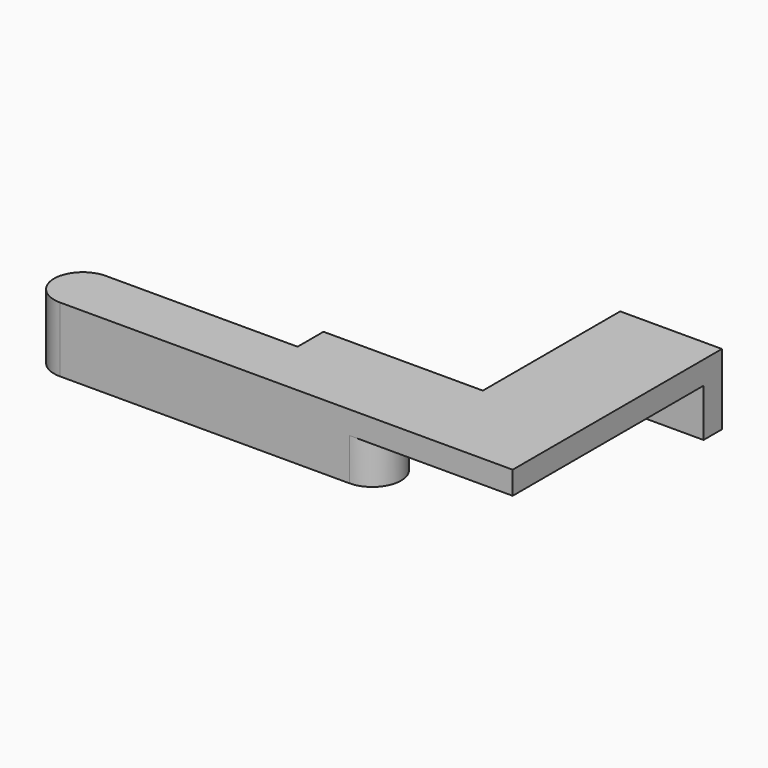
from build123d import *

# Parameters (mm, degrees)
F1_DEPTH = 4.6482
F2_W     = 11.2398419182
F2_H     = 2.54
F3_DEPTH = 2.54
F4_DEPTH = 5.2832


with BuildPart() as f1:
    # F0 (on Top) → F1 (new body)
    with BuildSketch(Plane.XY):
        with BuildLine():
            ThreePointArc((0, 6.35), (-3.175, 3.175), (0, 0))
            Line((0, 0), (31.9786, 0))
            ThreePointArc((31.9786, 0), (35.1536, 3.175), (31.9786, 6.35))
            Line((31.9786, 6.35), (0, 6.35))
        make_face()
    extrude(amount=F1_DEPTH)

    # F2 (on face) → F3 (join)
    with BuildSketch(Plane.XY.offset(4.6482)):
        Polygon((38.7858, 9.9314), (38.7858, 0), (50.0256419182, 0), (50.0256419182, 26.3525), (38.7858, 26.3525), align=None)
        with BuildLine():
            Line((31.9786, 0), (35.1536, 0))
            Line((35.1536, 0), (38.7858, 0))
            Line((38.7858, 0), (38.7858, 9.9314))
            Line((38.7858, 9.9314), (35.1536, 9.9314))
            Line((35.1536, 9.9314), (21.18106, 9.9314))
            Line((21.18106, 9.9314), (21.18106, 6.35))
            Line((21.18106, 6.35), (31.9786, 6.35))
            ThreePointArc((31.9786, 6.35), (35.1536, 3.175), (31.9786, 0))
        make_face()
        with BuildLine():
            Line((21.18106, 0), (31.9786, 0))
            ThreePointArc((31.9786, 0), (35.1536, 3.175), (31.9786, 6.35))
            Line((31.9786, 6.35), (21.18106, 6.35))
            Line((21.18106, 6.35), (21.18106, 0))
        make_face()
        with Locations((44.4057209591, 27.6225)):
            Rectangle(F2_W, F2_H)
        with BuildLine():
            Line((0, 0), (21.18106, 0))
            Line((21.18106, 0), (21.18106, 6.35))
            Line((21.18106, 6.35), (0, 6.35))
            ThreePointArc((0, 6.35), (-3.175, 3.175), (0, 0))
        make_face()
    extrude(amount=F3_DEPTH)

    # F2 (on face) → F4 (join)
    with BuildSketch(Plane.XY.offset(4.6482)):
        with Locations((44.4057209591, 27.6225)):
            Rectangle(F2_W, F2_H)
    extrude(amount=-F4_DEPTH)


solid = f1.part
